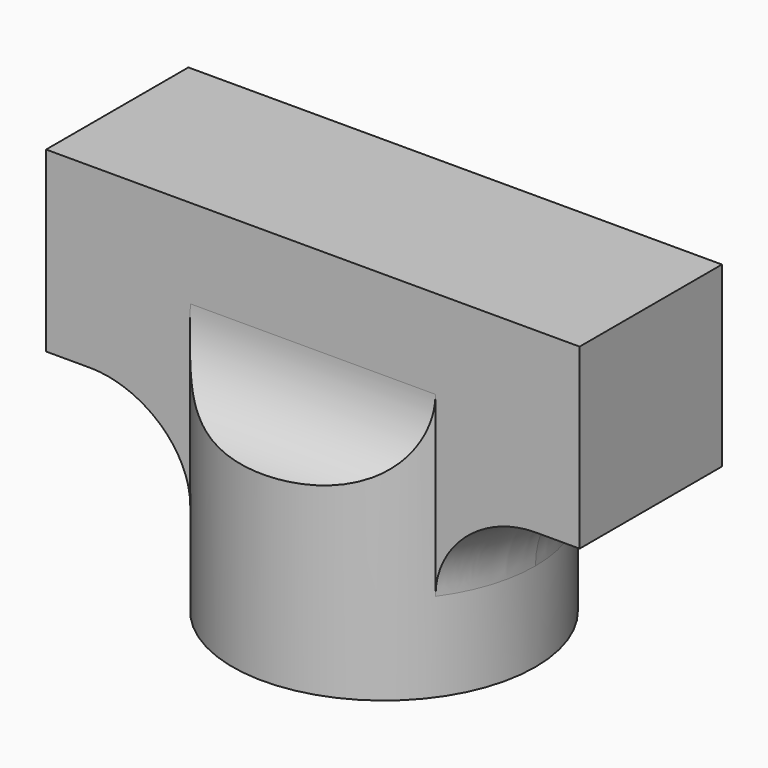
from build123d import *

# Parameters (mm, degrees)
F0_R         = 8.5154328933
F0_W         = 7.8
F0_H         = 7.8
F1_DEPTH     = 10
F2_W         = 7.8
F2_H         = 7.8
F3_DEPTH     = 10
F4_T4_DEPTH  = 38.7858764479
F4_S5_R      = 8.5154328933
F4_T6_DEPTH  = 21
F4_T10_DEPTH = 38.7858764479
F4_S11_R     = 8.5154328933
F4_T12_DEPTH = 21
F4_T16_ANGLE = 120.0675682876
F4_T21_ANGLE = 240.167490735
F4_T27_ANGLE = 120.0675682876


# Not quite as in the source:
# - a fillet or chamfer that OpenCascade refuses, or shapes differently, is made with other operations: its cross-section is extruded or revolved along the edge and cut away or added
# - two fillets or chamfers of one size are made in one step


with BuildPart() as f1:
    # F0 (on Top) → F1 (new body)
    with BuildSketch(Plane.XY):
        Circle(F0_R)
        Rectangle(F0_W, F0_H, mode=Mode.SUBTRACT)
    extrude(amount=F1_DEPTH)

    # F2 (on face) → F3 (join)
    with BuildSketch(Plane.XY.offset(10)):
        with BuildLine():
            Line((6.892938224, 5), (-6.892938224, 5))
            ThreePointArc((-6.892938224, 5), (-8.5154328933, 0), (-6.892938224, -5))
            Line((-6.892938224, -5), (6.892938224, -5))
            ThreePointArc((6.892938224, -5), (8.0996589509, -2.6283306942), (8.5154328933, 0))
            ThreePointArc((8.5154328933, 0), (8.0996589509, 2.6283306942), (6.892938224, 5))
        make_face()
        Rectangle(F2_W, F2_H, mode=Mode.SUBTRACT)
        with BuildLine():
            Line((-6.892938224, 5), (-15, 5))
            Line((-15, 5), (-15, -5))
            Line((-15, -5), (-6.892938224, -5))
            ThreePointArc((-6.892938224, -5), (-8.5154328933, 0), (-6.892938224, 5))
        make_face()
        with BuildLine():
            Line((15, 5), (6.892938224, 5))
            ThreePointArc((6.892938224, 5), (8.0996589509, 2.6283306942), (8.5154328933, 0))
            ThreePointArc((8.5154328933, 0), (8.0996589509, -2.6283306942), (6.892938224, -5))
            Line((6.892938224, -5), (15, -5))
            Line((15, -5), (15, 5))
        make_face()
        Rectangle(F2_W, F2_H)
    extrude(amount=F3_DEPTH)

    # F4: fillet of radius 5 on 5 edges, made by hand


with BuildPart() as f4_tool2:
    # F4_s3 → F4_t4 (new body)
    with BuildSketch(Plane.YZ.offset(-19.392938224)):
        with BuildLine():
            ThreePointArc((-10, 10), (-6.4644660941, 11.4644660941), (-5, 15))
            Line((-5, 15), (-5, 10))
            Line((-5, 10), (-10, 10))
        make_face()
    extrude(amount=F4_T4_DEPTH)

    # F4_s5 → F4_t6 (intersect, symmetric)
    with BuildSketch(Plane.XY.offset(12.5)):
        Circle(F4_S5_R)
    extrude(amount=F4_T6_DEPTH, both=True, mode=Mode.INTERSECT)


with BuildPart() as f1_1:
    add(f1.part)

    # F4_t1: union F4_tool2
    add(f4_tool2.part)


with BuildPart() as f4_tool8:
    # F4_s9 → F4_t10 (new body)
    with BuildSketch(Plane.YZ.offset(19.392938224)):
        with BuildLine():
            ThreePointArc((10, 10), (6.4644660941, 11.4644660941), (5, 15))
            Line((5, 15), (5, 10))
            Line((5, 10), (10, 10))
        make_face()
    extrude(amount=-F4_T10_DEPTH)

    # F4_s11 → F4_t12 (intersect, symmetric)
    with BuildSketch(Plane.XY.offset(12.5)):
        Circle(F4_S11_R)
    extrude(amount=F4_T12_DEPTH, both=True, mode=Mode.INTERSECT)


with BuildPart() as f1_2:
    add(f1_1.part)

    # F4_t7: union F4_tool8
    add(f4_tool8.part)


with BuildPart() as f4_tool14:
    # F4_s15 → F4_t16 (revolve)
    with BuildSketch(Plane(origin=(0, 0, 0), x_dir=(0, 0, 1), z_dir=(-0.8654351572, 0.5010209464, 0))):
        with BuildLine():
            ThreePointArc((5, -8.5154328933), (8.5355339059, -9.9798989873), (10, -13.5154328933))
            Line((10, -13.5154328933), (10, -8.5154328933))
            Line((10, -8.5154328933), (5, -8.5154328933))
        make_face()
    revolve(axis=Axis((0, 0, 10), (0, 0, 1)), revolution_arc=F4_T16_ANGLE)

    split(bisect_by=Plane.XZ.offset(5), keep=Keep.BOTTOM)


with BuildPart() as f1_3:
    add(f1_2.part)

    # F4_t13: union F4_tool14
    add(f4_tool14.part)


with BuildPart() as f4_tool19:
    # F4_s20 → F4_t21 (revolve)
    with BuildSketch(Plane(origin=(0, 0, 0), x_dir=(0, 0, 1), z_dir=(0.8652936628, -0.5012652762, 0))):
        with BuildLine():
            ThreePointArc((5, -8.5154328933), (8.5355339059, -9.9798989873), (10, -13.5154328933))
            Line((10, -13.5154328933), (10, -8.5154328933))
            Line((10, -8.5154328933), (5, -8.5154328933))
        make_face()
    revolve(axis=Axis((0, 0, 10), (0, 0, 1)), revolution_arc=F4_T21_ANGLE)

    split(bisect_by=Plane.XZ.offset(-5), keep=Keep.TOP)

    split(bisect_by=Plane.XZ.offset(5), keep=Keep.BOTTOM)


with BuildPart() as f1_4:
    add(f1_3.part)

    # F4_t18: union F4_tool19
    add(f4_tool19.part)


with BuildPart() as f4_tool25:
    # F4_s26 → F4_t27 (revolve)
    with BuildSketch(Plane.XZ):
        with BuildLine():
            ThreePointArc((8.5154328933, 5), (9.9798989873, 8.5355339059), (13.5154328933, 10))
            Line((13.5154328933, 10), (8.5154328933, 10))
            Line((8.5154328933, 10), (8.5154328933, 5))
        make_face()
    revolve(axis=Axis((0, 0, 10), (0, 0, 1)), revolution_arc=F4_T27_ANGLE)

    split(bisect_by=Plane.XZ.offset(-5), keep=Keep.TOP)


with BuildPart() as f1_5:
    add(f1_4.part)

    # F4_t24: union F4_tool25
    add(f4_tool25.part)


solid = f1_5.part
